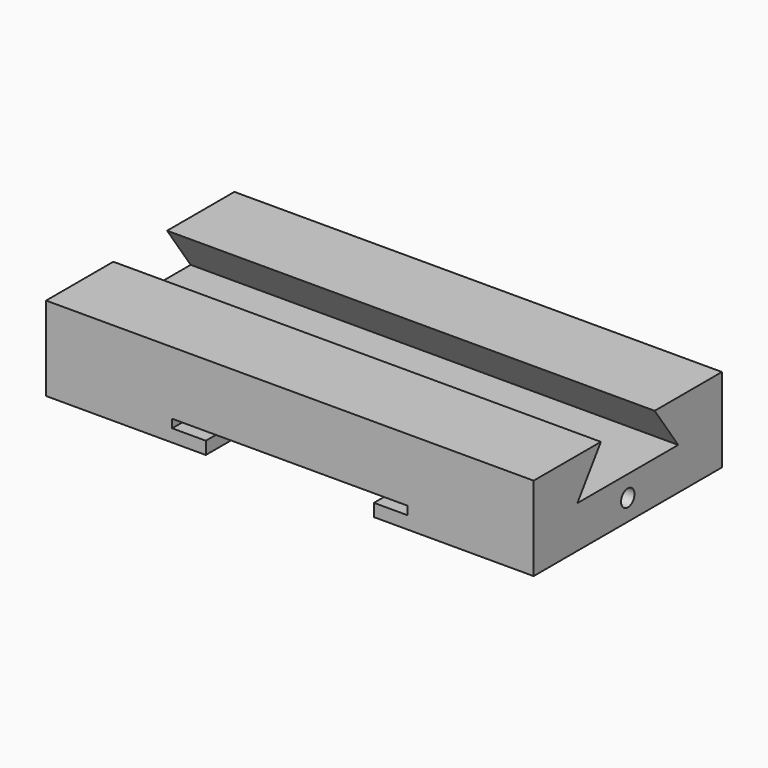
from build123d import *

# Parameters (mm, degrees)
F1_DEPTH  = 56
F3_DEPTH  = 116
F5_D      = 12
F5_DEPTH  = 5
F5_TIP    = 3.6051637142
F7_D      = 4
F7_DEPTH  = 6
F7_TIP    = 1.2017212381
F9_D      = 4
F9_DEPTH  = 6
F9_TIP    = 1.2017212381
F11_DEPTH = 56.001
F13_D     = 3
F13_DEPTH = 4
F13_TIP   = 0.9012909285


# Not quite as in the source:
# - a feature names something its author has since deleted; it is built from what else it names


with BuildPart() as f1:
    # F0 (on Front) → F1 (new body)
    with BuildSketch(Plane.XZ):
        Polygon((1.5, 0), (2, 2), (12, 2), (12.5, 0), (58, 0), (58, 20), (-58, 20), (-58, 0), (-12.5, 0), (-12, 2), (-2, 2), (-1.5, 0), (0, 0), align=None)
    extrude(amount=F1_DEPTH)

    # F2 (on face) → F3 (cut, through all)
    with BuildSketch(Plane(origin=(-58, 0, 0), x_dir=(0, -1, 0), z_dir=(-1, 0, 0))):
        Polygon((28, 20), (20.0020753821, 20), (13, 10), (28, 10), align=None)
        Polygon((35.9979246179, 20), (28, 20), (28, 10), (43, 10), align=None)
    extrude(amount=-F3_DEPTH, mode=Mode.SUBTRACT)

    # F5
    with Locations(Plane.XY.offset(10)):
        with Locations((0, -28)):
            Hole(F5_D / 2, depth=F5_DEPTH)
            with Locations((0, 0, -(F5_DEPTH + F5_TIP / 2))):  # 118° drill point
                Cone(0, F5_D / 2, F5_TIP, mode=Mode.SUBTRACT)

    # F7
    with Locations(Plane(origin=(-58, 0, 0), x_dir=(0, -1, 0), z_dir=(-1, 0, 0))):
        with Locations((28, 5)):
            Hole(F7_D / 2, depth=F7_DEPTH)
            with Locations((0, 0, -(F7_DEPTH + F7_TIP / 2))):  # 118° drill point
                Cone(0, F7_D / 2, F7_TIP, mode=Mode.SUBTRACT)

    # F9
    with Locations(Plane.YZ.offset(58)):
        with Locations((-28, 5)):
            Hole(F9_D / 2, depth=F9_DEPTH)
            with Locations((0, 0, -(F9_DEPTH + F9_TIP / 2))):  # 118° drill point
                Cone(0, F9_D / 2, F9_TIP, mode=Mode.SUBTRACT)

    # F10 (on face) → F11 (cut, through all)
    with BuildSketch(Plane.XZ.offset(56)):
        Polygon((12.5, 0), (20, 0), (20, 3), (28, 3), (28, 5), (20, 5), (0, 5), (0, 0), (1.5, 0), (2, 2), (12, 2), align=None)
        Polygon((-1.5, 0), (0, 0), (0, 5), (-20, 5), (-28, 5), (-28, 3), (-20, 3), (-20, 0), (-12.5, 0), (-12, 2), (-2, 2), align=None)
    extrude(amount=-F11_DEPTH, mode=Mode.SUBTRACT)

    # F13
    with Locations(Plane(origin=(0, 0, 0), x_dir=(1, 0, 0), z_dir=(0, 0, -1))):
        with Locations((-24, 46), (24, 46), (24, 10), (-24, 10)):
            Hole(F13_D / 2, depth=F13_DEPTH)
            with Locations((0, 0, -(F13_DEPTH + F13_TIP / 2))):  # 118° drill point
                Cone(0, F13_D / 2, F13_TIP, mode=Mode.SUBTRACT)


solid = f1.part
